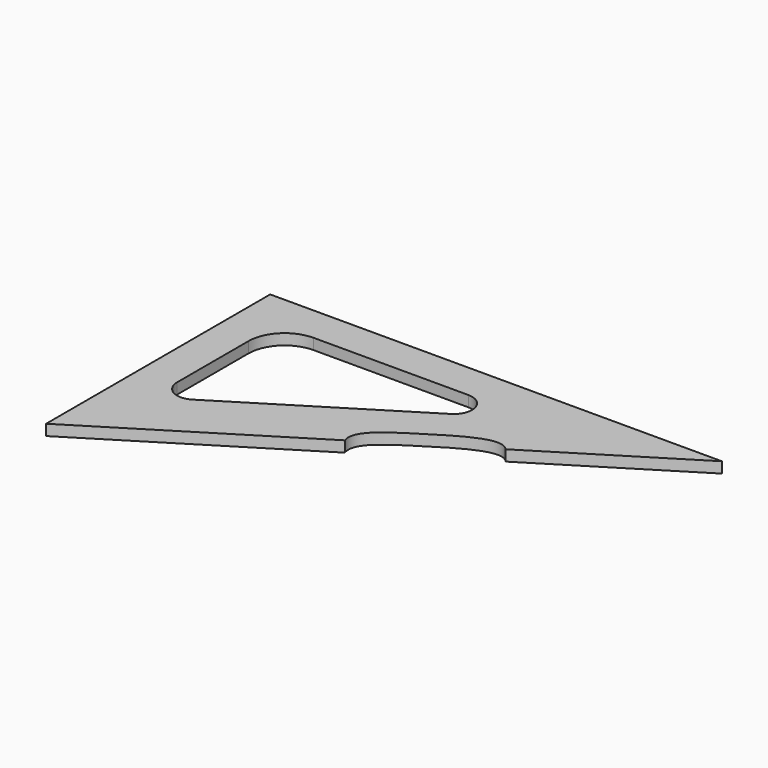
from build123d import *

# Parameters (mm, degrees)
F1_DEPTH = 6


with BuildPart() as f1:
    # F0 (on Top) → F1 (new body)
    with BuildSketch(Plane.XY):
        with BuildLine():
            Line((250, 0), (0, 0))
            Line((0, 0), (0, -155))
            Line((0, -155), (110.4873499226, -86.497843048))
            add(Edge.make_bspline(
                [(110.4873499226, -86.497843048), (107.2843735439, -77.0023074484), (131.9373436968, -61.4037722235), (163.3322021719, -41.7004632777), (169.9805383425, -49.6120662277)],
                knots=[0, 0, 0, 0, 0.2195299732, 0.4558974308, 0.4558974308, 0.4558974308, 0.4558974308], degree=3))
            Line((169.9805383425, -49.6120662277), (250, 0))
        make_face()
        with BuildLine():
            Line((20, -89.3357885437), (20, -40))
            ThreePointArc((20, -40), (25.8578643763, -25.8578643763), (40, -20))
            Line((40, -20), (125.702884748, -20))
            ThreePointArc((125.702884748, -20), (135.3203238346, -27.2604990574), (130.9722814366, -38.4990269171))
            Line((130.9722814366, -38.4990269171), (35.2693966886, -97.8348154609))
            ThreePointArc((35.2693966886, -97.8348154609), (25.1365632977, -98.0734646331), (20, -89.3357885437))
        make_face(mode=Mode.SUBTRACT)
    extrude(amount=-F1_DEPTH)


solid = f1.part
